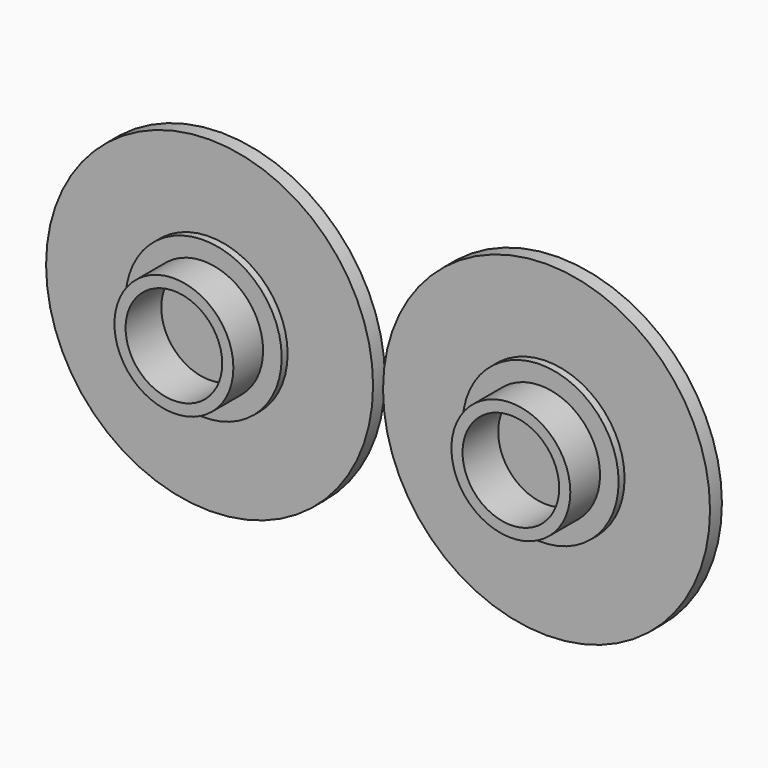
from build123d import *

# Parameters (mm, degrees)
F0_R     = 11
F0_R_2   = 5.25
F1_DEPTH = 1
F0_R_3   = 3.25
F0_R_4   = 4
F2_DEPTH = 1.5
F3_DEPTH = 4


with BuildPart() as f1:
    # F0 (on Front) → F1 (new body)
    with BuildSketch(Plane.XZ):
        Circle(F0_R)
        Circle(F0_R_2, mode=Mode.SUBTRACT)
    extrude(amount=F1_DEPTH)

    # F0 (on Front) → F2 (join)
    with BuildSketch(Plane.XZ):
        Circle(F0_R_2)
        Circle(F0_R_4, mode=Mode.SUBTRACT)
    extrude(amount=F2_DEPTH)


with BuildPart() as f1b:
    # F0 (on Front) → F1, piece 2 (new body)
    with BuildSketch(Plane.XZ):
        Circle(F0_R_3)
    extrude(amount=F1_DEPTH)


with BuildPart() as f1c:
    # F0 (on Front) → F1, piece 3 (new body)
    with BuildSketch(Plane.XZ):
        with Locations((-22.6695239544, 0)):
            Circle(F0_R)
        with Locations((-22.6695239544, 0)):
            Circle(F0_R_2, mode=Mode.SUBTRACT)
    extrude(amount=F1_DEPTH)


with BuildPart() as f1d:
    # F0 (on Front) → F1, piece 4 (new body)
    with BuildSketch(Plane.XZ):
        with Locations((-22.6695239544, 0)):
            Circle(F0_R_3)
    extrude(amount=F1_DEPTH)


with BuildPart() as f2:
    # F0 (on Front) → F2, piece 2 (new body)
    with BuildSketch(Plane.XZ):
        with Locations((-22.6695239544, 0)):
            Circle(F0_R_2)
        with Locations((-22.6695239544, 0)):
            Circle(F0_R_4, mode=Mode.SUBTRACT)
    extrude(amount=F2_DEPTH)


with BuildPart() as f3:
    # F0 (on Front) → F3 (new body)
    with BuildSketch(Plane.XZ):
        Circle(F0_R_4)
        Circle(F0_R_3, mode=Mode.SUBTRACT)
    extrude(amount=F3_DEPTH)


with BuildPart() as f3b:
    # F0 (on Front) → F3, piece 2 (new body)
    with BuildSketch(Plane.XZ):
        with Locations((-22.6695239544, 0)):
            Circle(F0_R_4)
        with Locations((-22.6695239544, 0)):
            Circle(F0_R_3, mode=Mode.SUBTRACT)
    extrude(amount=F3_DEPTH)


solid = Compound([f1.part, f1b.part, f1c.part, f1d.part, f2.part, f3.part, f3b.part])
